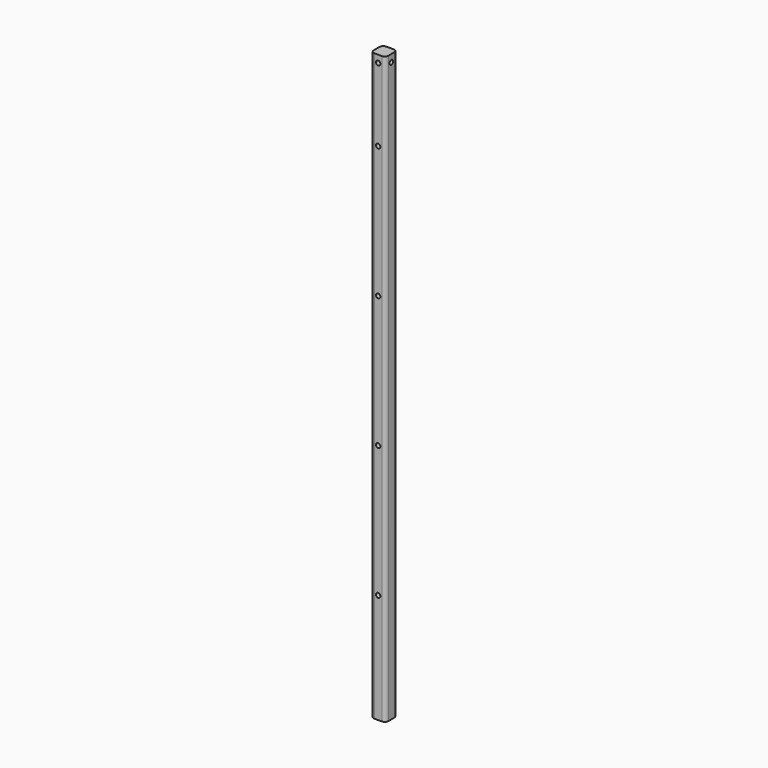
from build123d import *

# Parameters (mm, degrees)
F1_DEPTH = 1016
F4_DEPTH = 25.4
F2_R     = 3.81
F5_DEPTH = 25.4
F6_DEPTH = 25.4


# Not quite as in the source:
# - a feature names something its author has since deleted; it is built from what else it names


with BuildPart() as f1:
    # F0 (on Top) → F1 (new body)
    with BuildSketch(Plane.XY):
        with BuildLine():
            ThreePointArc((12.7, 6.35), (10.8401280605, 10.8401280605), (6.35, 12.7))
            Line((6.35, 12.7), (-6.35, 12.7))
            ThreePointArc((-6.35, 12.7), (-10.8401280605, 10.8401280605), (-12.7, 6.35))
            Line((-12.7, 6.35), (-12.7, -6.35))
            ThreePointArc((-12.7, -6.35), (-10.8401280605, -10.8401280605), (-6.35, -12.7))
            Line((-6.35, -12.7), (6.35, -12.7))
            ThreePointArc((6.35, -12.7), (10.8401280605, -10.8401280605), (12.7, -6.35))
            Line((12.7, -6.35), (12.7, 6.35))
        make_face()
    extrude(amount=F1_DEPTH)

    # F3 (on face) → F4 (cut)
    with BuildSketch(Plane.YZ.offset(12.7)):
        with BuildLine():
            ThreePointArc((3.81, 1003.3), (2.6940768363, 1005.9940768363), (0, 1007.11))
            ThreePointArc((0, 1007.11), (-2.6940768363, 1000.6059231637), (3.81, 1003.3))
        make_face()
    extrude(amount=-F4_DEPTH, mode=Mode.SUBTRACT)

    # F2 (on face) → F5 (cut)
    with BuildSketch(Plane.XZ.offset(12.7)):
        with BuildLine():
            ThreePointArc((3.81, 1003.3), (2.6940768363, 1005.9940768363), (0, 1007.11))
            ThreePointArc((0, 1007.11), (-2.6940768363, 1000.6059231637), (3.81, 1003.3))
        make_face()
        with Locations((0, 876.3)):
            Circle(F2_R)
        with Locations((0, 647.7)):
            Circle(F2_R)
        with Locations((0, 419.1)):
            Circle(F2_R)
    extrude(amount=-F5_DEPTH, mode=Mode.SUBTRACT)

    # F2 (on face) → F6 (cut)
    with BuildSketch(Plane.XZ.offset(12.7)):
        with Locations((0, 190.5)):
            Circle(F2_R)
    extrude(amount=-F6_DEPTH, mode=Mode.SUBTRACT)


solid = f1.part
